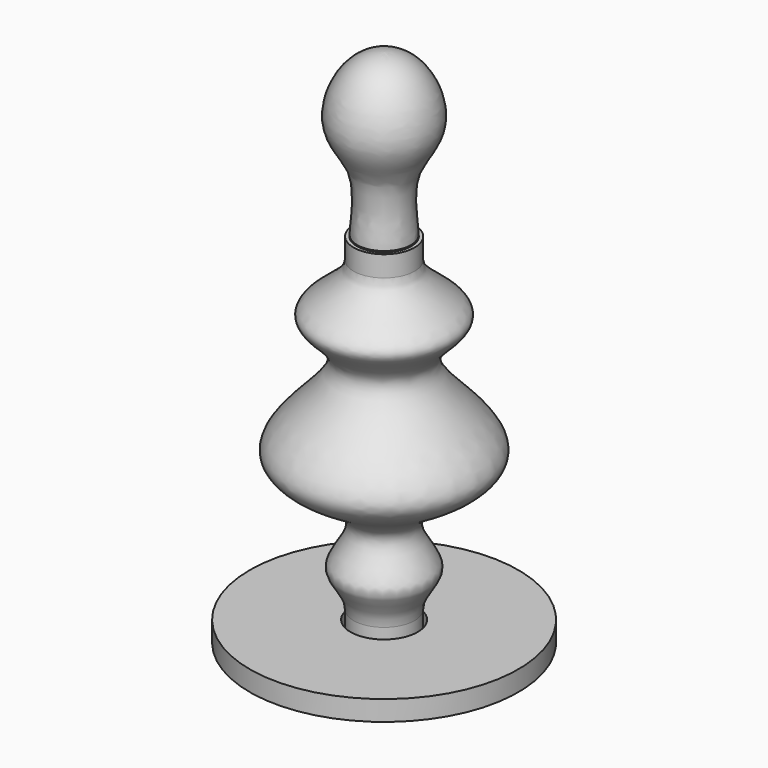
from build123d import *

# Parameters (mm, degrees)
F0_W = 75
F0_H = 15
F4_T = -2.5


# Not quite as in the source:
# - a feature of the source that left no trace in its solid (it failed there, or was rolled back) is left out


with BuildPart() as f1:
    # F0 (on Front) → F1 (revolve)
    with BuildSketch(Plane.XZ):
        with Locations((-62.5, 7.5)):
            Rectangle(F0_W, F0_H)
    revolve(axis=Axis((0, 0, 28.5546835512), (0, 0, 1)))


with BuildPart() as f3:
    # F2 (on Front) → F3 (revolve)
    with BuildSketch(Plane.XZ):
        with BuildLine():
            Line((-22.7263234556, 21.7216983438), (-22.7263234556, 0))
            Line((-22.7263234556, 0), (0, 0))
            Line((0, 0), (0, 266.2498950958))
            Line((0, 266.2498950958), (-22.7263234556, 266.2498950958))
            Line((-22.7263234556, 266.2498950958), (-22.7263234556, 250.7138252258))
            add(Edge.make_bspline(
                [(-22.7263234556, 250.7138252258), (-22.7263234556, 237.0224211611), (-75.2576582833, 216.0218915756), (-3.8676634027, 185.8192369168), (-114.1082361223, 119.3624638974), (1.4196364649, 87.636575241), (-47.0539357888, 48.5750019051), (-22.7263234556, 34.5982177026), (-22.7263234556, 21.7216983438)],
                knots=[0, 0, 0, 0, 0.166187118, 0.31235361, 0.5222344792, 0.7219499539, 0.8632624919, 1, 1, 1, 1], degree=3))
        make_face()
    revolve(axis=Axis((0, 0, 133.1249475479), (0, 0, 1)))

    # F4
    f4_openings = [f3.faces().sort_by_distance(p)[0] for p in [
        (0, 0, 266.249895),
        (0, 0, 0),
    ]]
    offset(amount=F4_T, openings=f4_openings)


with BuildPart() as f10:
    # F9 (on Front) → F10 (revolve)
    with BuildSketch(Plane.XZ):
        with BuildLine():
            Line((-20, 267), (0, 267))
            Line((0, 267), (0, 387))
            add(Edge.make_bspline(
                [(0, 387), (-23.7923519673, 387), (-48.2496290638, 338.8623447177), (-13.3288953811, 311.1294410668), (-20, 277.4873915765), (-20, 267)],
                knots=[0, 0, 0, 0, 0.3744713465, 0.6848860157, 1, 1, 1, 1], degree=3))
        make_face()
    revolve(axis=Axis((0, 0, 327), (0, 0, 1)))


solid = Compound([f1.part, f3.part, f10.part])
